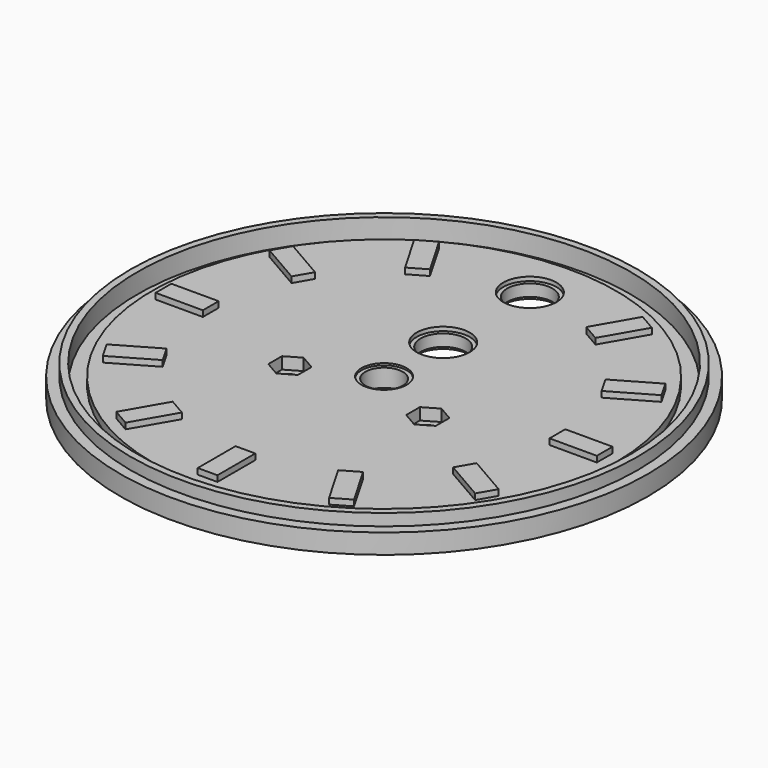
from build123d import *

# Parameters (mm, degrees)
F0_R              = 67
F1_DEPTH          = 2.5
F2_R              = 64.375
F2_R_2            = 62.625
F3_DEPTH          = 3
F2_R_3            = 58.875
F4_DEPTH          = 2
F5_R              = 4.75
F5_R_2            = 5.75
F5_R_3            = 2.1
F6_DEPTH          = 25
F7_R              = 5.75
F7_R_2            = 4.75
F8_DEPTH          = 0.5
F7_R_3            = 6.75
F9_DEPTH          = 1
F7_R_4            = 2.1
F10_DEPTH         = 3
F11_R             = 6.75
F11_R_2           = 5.75
F12_DEPTH         = 1
F13_W             = 5
F13_H             = 12
F14_DEPTH         = 1.5
F14_COPIES_COUNT  = 6
F14_COPIES_ANGLE  = 150
F14_COPIES1_COUNT = 6
F14_COPIES1_ANGLE = 150


# Not quite as in the source:
# - a feature of the source that left no trace in its solid (it failed there, or was rolled back) is left out
# - a pattern or mirror of a feature is missing from the dataset's text; its kind, count and spacing are read off the source's solid


with BuildPart() as f1:
    # F0 (on Top) → F1 (new body, symmetric)
    with BuildSketch(Plane.XY):
        Circle(F0_R)
    extrude(amount=F1_DEPTH, both=True)

    # F2 (on face) → F3 (join)
    with BuildSketch(Plane.XY.offset(2.5)):
        Circle(F2_R)
        Circle(F2_R_2, mode=Mode.SUBTRACT)
    extrude(amount=F3_DEPTH)

    # F2 (on face) → F4 (cut)
    with BuildSketch(Plane.XY.offset(2.5)):
        Circle(F2_R_2)
        Circle(F2_R_3, mode=Mode.SUBTRACT)
    extrude(amount=-F4_DEPTH, mode=Mode.SUBTRACT)

    # F5 (on face) → F6 (cut)
    with BuildSketch(Plane.XY.offset(2.5)):
        Circle(F5_R)
        with Locations((0, 18.75)):
            Circle(F5_R_2)
        with Locations((0, 46.25)):
            Circle(F5_R_2)
        with Locations((17.5, -8)):
            Circle(F5_R_3)
        with Locations((-17.5, -8)):
            Circle(F5_R_3)
    extrude(amount=-F6_DEPTH, mode=Mode.SUBTRACT)

    # F7 (on face) → F8 (cut)
    with BuildSketch(Plane.XY.offset(2.5)):
        Circle(F7_R)
        Circle(F7_R_2, mode=Mode.SUBTRACT)
    extrude(amount=-F8_DEPTH, mode=Mode.SUBTRACT)

    # F7 (on face) → F9 (cut)
    with BuildSketch(Plane.XY.offset(2.5)):
        with Locations((0, 18.75)):
            Circle(F7_R_3)
        with Locations((0, 18.75)):
            Circle(F7_R, mode=Mode.SUBTRACT)
        with Locations((0, 46.25)):
            Circle(F7_R_3)
        with Locations((0, 46.25)):
            Circle(F7_R, mode=Mode.SUBTRACT)
    extrude(amount=-F9_DEPTH, mode=Mode.SUBTRACT)

    # F7 (on face) → F10 (cut)
    with BuildSketch(Plane.XY.offset(2.5)):
        Polygon((-13.75, -10.1650635095), (-13.75, -5.8349364905), (-17.5, -3.6698729811), (-21.25, -5.8349364905), (-21.25, -10.1650635095), (-17.5, -12.3301270189), align=None)
        with Locations((-17.5, -8)):
            Circle(F7_R_4, mode=Mode.SUBTRACT)
        Polygon((21.25, -10.1650635095), (21.25, -5.8349364905), (17.5, -3.6698729811), (13.75, -5.8349364905), (13.75, -10.1650635095), (17.5, -12.3301270189), align=None)
        with Locations((17.5, -8)):
            Circle(F7_R_4, mode=Mode.SUBTRACT)
    extrude(amount=-F10_DEPTH, mode=Mode.SUBTRACT)

    # F11 (on face) → F12 (cut)
    with BuildSketch(Plane(origin=(0, 0, -2.5), x_dir=(1, 0, 0), z_dir=(0, 0, -1))):
        with Locations((0, -18.75)):
            Circle(F11_R)
        with Locations((0, -18.75)):
            Circle(F11_R_2, mode=Mode.SUBTRACT)
        with Locations((0, -46.25)):
            Circle(F11_R)
        with Locations((0, -46.25)):
            Circle(F11_R_2, mode=Mode.SUBTRACT)
    extrude(amount=-F12_DEPTH, mode=Mode.SUBTRACT)

    # F13 (on face) → F14 (join)
    with BuildSketch(Plane.XY.offset(2.5)):
        with Locations((0, -50)):
            Rectangle(F13_W, F13_H)
    f14 = extrude(amount=F14_DEPTH)

    # F14_copies: F14 ×6 about axis
    f14_copies_axis = Axis((0, 0, 0), (0, 0, 1))
    for i in range(1, F14_COPIES_COUNT):
        add(f14.rotate(f14_copies_axis, i * F14_COPIES_ANGLE / (F14_COPIES_COUNT - 1)))

    # F14_copies1: F14 ×6 about axis
    f14_copies1_axis = Axis((0, 0, 0), (0, 0, -1))
    for i in range(1, F14_COPIES1_COUNT):
        add(f14.rotate(f14_copies1_axis, i * F14_COPIES1_ANGLE / (F14_COPIES1_COUNT - 1)))


solid = f1.part
